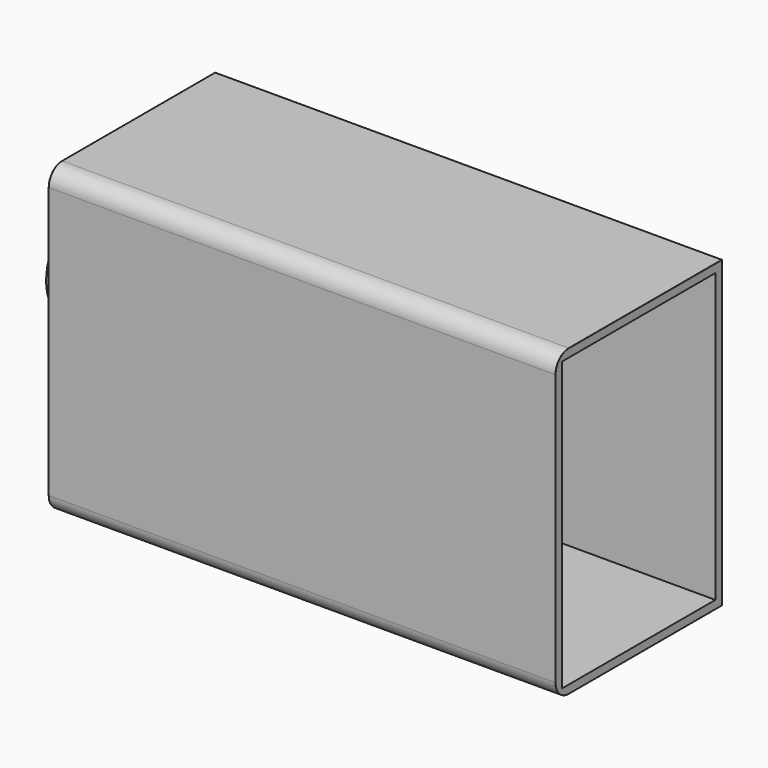
from build123d import *

# Parameters (mm, degrees)
F0_W     = 60.8845241368
F0_H     = 36.5624986589
F1_DEPTH = 25
F2_T     = -1
F3_R     = 5.8019318328
F3_R_2   = 5.7407936272
F4_DEPTH = 5.9
F5_DEPTH = 11.4
F6_T     = -2.5
F9_D     = 2
F10_R    = 2
F11_R    = 0.0241421356
F12_R    = 0.0241421356


# Not quite as in the source:
# - a feature of the source that left no trace in its solid (it failed there, or was rolled back) is left out


with BuildPart() as f1:
    # F0 (on Front) → F1 (new body)
    with BuildSketch(Plane.XZ):
        with Locations((-30.4422620684, -18.2812493294)):
            Rectangle(F0_W, F0_H)
    extrude(amount=F1_DEPTH)

    # F2
    f2_openings = [f1.faces().sort_by_distance(p)[0] for p in [
        (0, -12.5, -18.281249),
    ]]
    offset(amount=F2_T, openings=f2_openings)

    # F3 (on face) → F4 (join)
    with BuildSketch(Plane(origin=(-60.8845241368, 0, 0), x_dir=(0, -1, 0), z_dir=(-1, 0, 0))):
        with Locations((12.2040687129, -16.6244860739)):
            Circle(F3_R)
        with Locations((12.2040687129, -16.6244860739)):
            Circle(F3_R_2, mode=Mode.SUBTRACT)
    extrude(amount=F4_DEPTH)

    # F5 (add): a face of the model
    f5_faces = [f1.faces().sort_by_distance(p)[0] for p in [
        (-60.8845241368, -12.2040687129, -16.6244860739),
    ]]
    extrude(f5_faces, amount=-F5_DEPTH)

    # F6
    f6_openings = [f1.faces().sort_by_distance(p)[0] for p in [
        (-49.484524, -12.204069, -16.624486),
    ]]
    offset(amount=F6_T, openings=f6_openings)

    # F9 (through all)
    with Locations(Plane(origin=(-60.8845241368, 0, 0), x_dir=(0, -1, 0), z_dir=(-1, 0, 0))):
        with Locations((12.2040687129, -16.6244860739)):
            Hole(F9_D / 2)

    # F10
    f10_edges = [f1.edges().sort_by_distance(p)[0] for p in [
        (-30.442262, -25, -36.562499),
        (-30.442262, -25, 0),
    ]]
    fillet(f10_edges, radius=F10_R)

    # F11
    f11_edges = [f1.edges().sort_by_distance(p)[0] for p in [
        (-30.442262, 0, -36.562499),
        (-30.442262, 0, 0),
    ]]
    fillet(f11_edges, radius=F11_R)

    # F12
    f12_edges = [f1.edges().sort_by_distance(p)[0] for p in [
        (-30.442262, -0.024142, -36.562499),
        (-30.442262, 0, -0.024142),
        (0, 0, -18.281249),
        (-60.884524, 0, -18.281249),
        (0, -11.512071, 0),
        (-60.884524, -11.512071, 0),
        (0, -11.512071, -36.562499),
        (0, -0.007071, -36.555428),
        (0, -24.414214, -35.976712),
        (0, -25, -18.281249),
        (0, -0.007071, -0.007071),
        (0, -24.414214, -0.585786),
        (-60.884524, -0.007071, -0.007071),
        (-60.884524, -24.414214, -0.585786),
        (-60.884524, -25, -18.281249),
        (-60.884524, -0.007071, -36.555428),
        (-60.884524, -24.414214, -35.976712),
        (-60.884524, -11.512071, -36.562499),
    ]]
    fillet(f12_edges, radius=F12_R)


solid = f1.part
